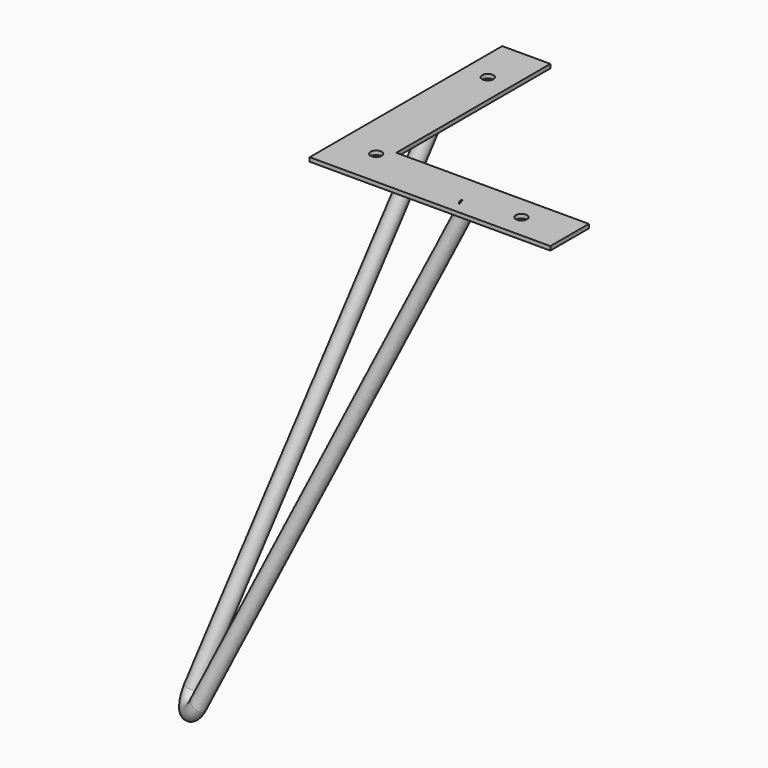
from build123d import *

# Parameters (mm, degrees)
F0_R     = 4.75
F0_R_2   = 3.5
F1_DEPTH = 2.5
F9_R     = 4.75


with BuildPart() as f1:
    # F0 (on Top) → F1 (new body)
    with BuildSketch(Plane.XY):
        Polygon((0, 150), (0, 0), (150, 0), (150, 10), (150, 30), (30, 30), (30, 150), (10, 150), align=None)
        with Locations((10, 10)):
            Circle(F0_R, mode=Mode.SUBTRACT)
        with Locations((23, 23)):
            Circle(F0_R_2, mode=Mode.SUBTRACT)
        with Locations((90, 10)):
            Circle(F0_R, mode=Mode.SUBTRACT)
        with Locations((120, 15)):
            Circle(F0_R_2, mode=Mode.SUBTRACT)
        with Locations((10, 90)):
            Circle(F0_R, mode=Mode.SUBTRACT)
        with Locations((15, 120)):
            Circle(F0_R_2, mode=Mode.SUBTRACT)
        with Locations((10, 10)):
            Circle(F0_R)
        with Locations((90, 10)):
            Circle(F0_R)
        with Locations((10, 90)):
            Circle(F0_R)
    extrude(amount=F1_DEPTH)

    # F10: sweep along a path in F7
    with BuildLine(Plane(origin=(42.039800995, 42.039800995, -25.8706467662), x_dir=(0.5521991294, -0.7613159594, -0.3398148488), z_dir=(-0.6483810685, -0.6483810685, 0.3990037344))) as f10_path:
        Line((-62.9964450532, 5.2409742566), (96.5428984083, -271.7818964901))
        ThreePointArc((96.5428984083, -271.7818964901), (108.8813288368, -276.0923992559), (114.9460414041, -264.5149832658))
        Line((114.9460414041, -264.5149832658), (42.084762048, 47.1687683098))
    # F9 (on face) → F10 (sweep)
    with BuildSketch(Plane(origin=(2.1613635589, 2.1613635589, 14.3803119238), x_dir=(0.9891341488, -0.021851066, -0.1453828274), z_dir=(0.1470157665, 0.1470157665, 0.9781476007))):
        with Locations((7.9247455466, 89.0003486068)):
            Circle(F9_R)
    sweep(path=f10_path.line)


solid = f1.part
